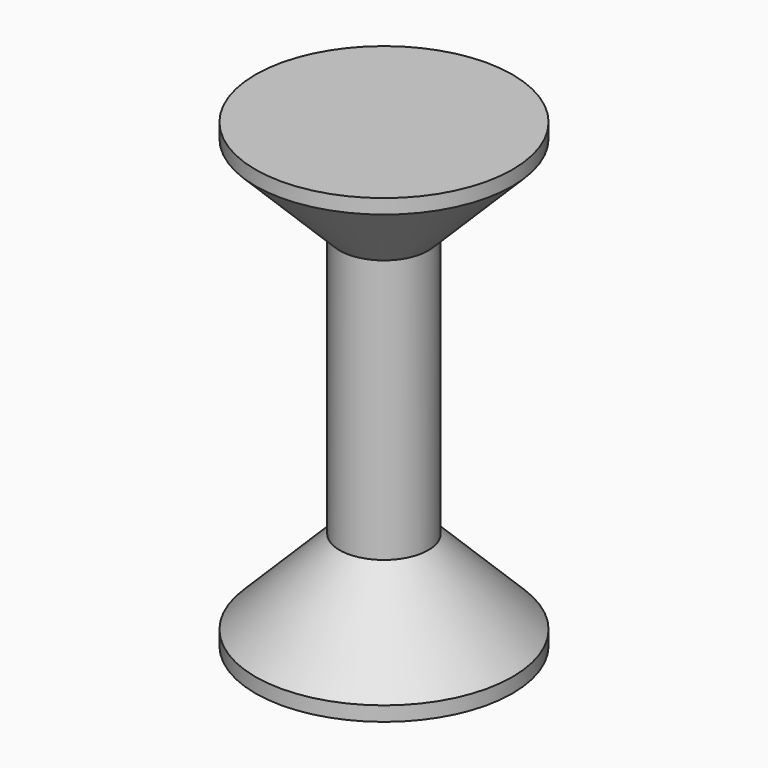
from build123d import *

# Parameters (mm, degrees)
F0_R         = 18.3771927797
F1_DEPTH     = 89.916
F2_R         = 53.2482574965
F2_R_2       = 18.3771927797
F3_DEPTH     = 5.588
F5_S5_R      = 53.2482574965
F5_T6_DEPTH  = 79
F5_S11_R     = 53.2482574965
F5_T12_DEPTH = 79


# Not quite as in the source:
# - a fillet or chamfer that OpenCascade refuses, or shapes differently, is made with other operations: its cross-section is extruded or revolved along the edge and cut away or added


with BuildPart() as f1:
    # F0 (on Top) → F1 (new body)
    with BuildSketch(Plane.XY):
        Circle(F0_R)
    extrude(amount=F1_DEPTH)

    # F2 (on face) → F3 (join)
    with BuildSketch(Plane.XY.offset(89.916)):
        Circle(F2_R)
        Circle(F2_R_2, mode=Mode.SUBTRACT)
        Circle(F2_R_2)
    extrude(amount=F3_DEPTH)

    # F4: F1 across plane


with BuildPart() as f1_1:
    add(f1.part)
    add(f1.part.mirror(Plane.XY))

    # F5: chamfer of 35.306 on 5 edges, made by hand


with BuildPart() as f5_tool2:
    # F5_s3 → F5_t4 (revolve)
    with BuildSketch(Plane.XZ):
        Polygon((53.6831927797, 89.916), (18.3771927797, 54.61), (18.3771927797, 89.916), align=None)
    revolve(axis=Axis((0, 0, 89.916), (0, 0, 1)))

    # F5_s5 → F5_t6 (intersect, symmetric)
    with BuildSketch(Plane.XY.offset(72.3)):
        Circle(F5_S5_R)
    extrude(amount=F5_T6_DEPTH, both=True, mode=Mode.INTERSECT)


with BuildPart() as f1_2:
    add(f1_1.part)

    # F5_t1: union F5_tool2
    add(f5_tool2.part)


with BuildPart() as f5_tool8:
    # F5_s9 → F5_t10 (revolve)
    with BuildSketch(Plane.XZ):
        Polygon((18.3771927797, -54.61), (53.6831927797, -89.916), (18.3771927797, -89.916), align=None)
    revolve(axis=Axis((0, 0, -89.916), (0, 0, 1)))

    # F5_s11 → F5_t12 (intersect, symmetric)
    with BuildSketch(Plane.XY.offset(-72.3)):
        Circle(F5_S11_R)
    extrude(amount=F5_T12_DEPTH, both=True, mode=Mode.INTERSECT)


with BuildPart() as f1_3:
    add(f1_2.part)

    # F5_t7: union F5_tool8
    add(f5_tool8.part)


solid = f1_3.part
